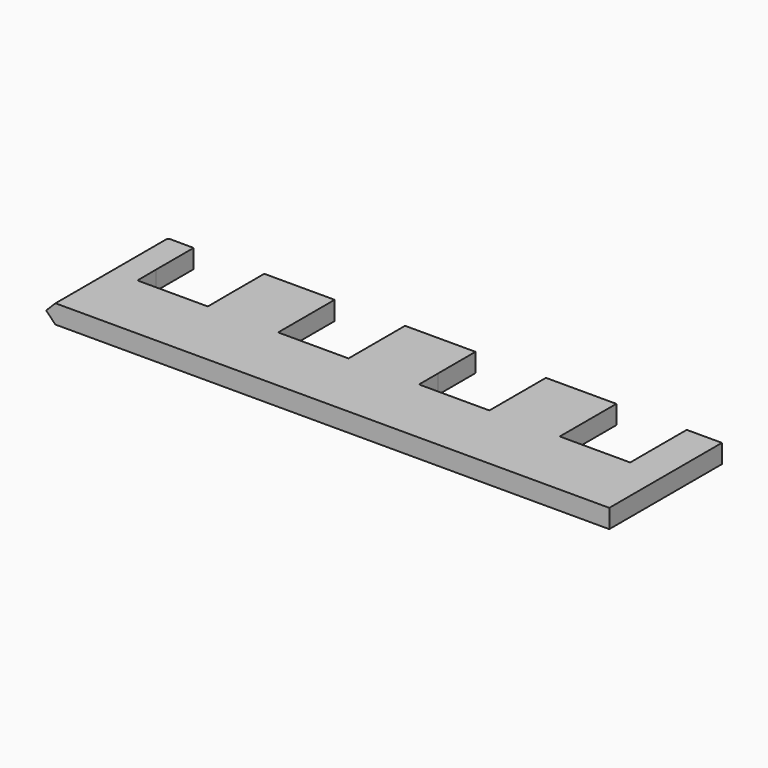
from build123d import *

# Parameters (mm, degrees)
F1_DEPTH = 4
F2_SIZE  = 2.3
F3_SIZE  = 1.99999


# Not quite as in the source:
# - a fillet or chamfer is up to 0.001 mm smaller than in the source, because OpenCascade refuses the exact size


with BuildPart() as f1:
    # F0 (on Top) → F1 (new body)
    with BuildSketch(Plane.XY):
        Polygon((-75.4356830697, -28.6679565907), (-75.4356830697, -30), (44.5643169303, -30), (44.5643169303, 0), (37.0643169303, 0), (37.0643169303, -10), (37.0643169303, -15.06), (22.0643169303, -15.06), (22.0643169303, -10), (22.0643169303, 0), (7.0643169303, 0), (7.0643169303, -10), (7.0643169303, -15.06), (-7.9356830697, -15.06), (-7.9356830697, -10), (-7.9491234598, 0), (-22.9491234598, 0), (-22.9491234598, -10), (-22.9491234598, -15.06), (-37.9491234598, -15.06), (-37.9491234598, -10), (-37.9491234598, 0), (-52.9491234598, 0), (-52.9491234598, -10), (-52.9229563225, -15.06), (-67.9233574687, -15.06), (-67.9491234598, -10.077570565), (-67.9491234598, -0.077570565), (-75.4356830697, 0), (-75.4356830697, -15.06), align=None)
    extrude(amount=F1_DEPTH)

    # F2
    f2_edges = [f1.edges().sort_by_distance(p)[0] for p in [
        (-75.435683, 0, 2),
    ]]
    chamfer(f2_edges, length=F2_SIZE)

    # F3 (size 2 in the source; OpenCascade refuses exactly that, so slightly less here)
    f3_edges = [f1.edges().sort_by_distance(p)[0] for p in [
        (-75.435683, -16.15, 0),
        (-75.435683, -16.15, 4),
    ]]
    chamfer(f3_edges, length=F3_SIZE)


solid = f1.part
